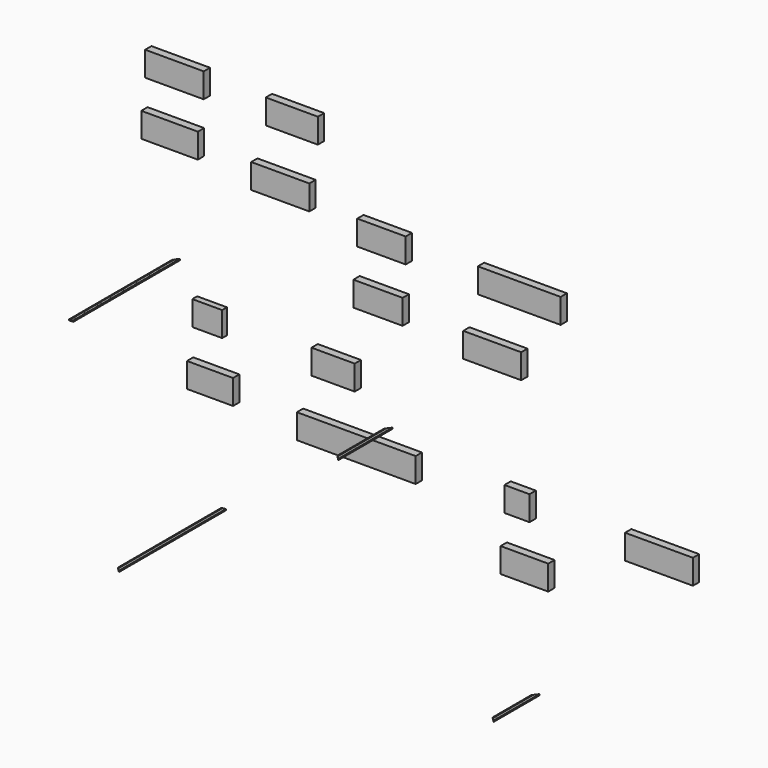
from build123d import *

# Parameters (mm, degrees)
F0_W        = 920.75
F0_H        = 387.35
F1_DEPTH    = 123.825
F0_W_2      = 889
F0_W_3      = 819.15
F0_W_4      = 914.4
F2_DEPTH    = 2101.85
F3_R        = 3.17499
F4_T1_DEPTH = 368.7891234188
F5_DEPTH    = 2101.85
F6_SIZE     = 69.84999
F0_W_5      = 762
F7_DEPTH    = 123.825
F0_W_6      = 1301.75
F0_W_7      = 774.7
F8_DEPTH    = 123.825
F0_W_8      = 911.225
F9_DEPTH    = 123.825
F0_W_9      = 679.45
F10_DEPTH   = 123.825
F0_W_10     = 469.9
F11_DEPTH   = 95.25
F0_W_11     = 723.9
F12_DEPTH   = 123.825
F0_W_12     = 1867.8652
F13_DEPTH   = 123.825
F0_W_13     = 393.7
F14_DEPTH   = 123.825
F0_W_14     = 1066.8
F15_DEPTH   = 123.825
F16_DEPTH   = 901.7
F17_SIZE    = 69.84999
F18_DEPTH   = 1060.45
F19_SIZE    = 69.84999
F0_W_15     = 749.3
F20_DEPTH   = 123.825


# Not quite as in the source:
# - a fillet or chamfer that OpenCascade refuses, or shapes differently, is made with other operations: its cross-section is extruded or revolved along the edge and cut away or added
# - a fillet or chamfer is up to 0.001 mm smaller than in the source, because OpenCascade refuses the exact size


with BuildPart() as f1:
    # F0 (on Front) → F1 (new body)
    with BuildSketch(Plane.XZ):
        with Locations((43.4228066687, 51.0344691575)):
            Rectangle(F0_W, F0_H)
    extrude(amount=F1_DEPTH)


with BuildPart() as f1b:
    # F0 (on Front) → F1, piece 2 (new body)
    with BuildSketch(Plane.XZ):
        with Locations((-33.3776168823, -813.8792926788)):
            Rectangle(F0_W_2, F0_H)
    extrude(amount=F1_DEPTH)


with BuildPart() as f1c:
    # F0 (on Front) → F1, piece 3 (new body)
    with BuildSketch(Plane.XZ):
        with Locations((1888.5462429047, 6.92840271)):
            Rectangle(F0_W_3, F0_H)
    extrude(amount=F1_DEPTH)


with BuildPart() as f1d:
    # F0 (on Front) → F1, piece 4 (new body)
    with BuildSketch(Plane.XZ):
        with Locations((1706.7899200439, -960.758965683)):
            Rectangle(F0_W_4, F0_H)
    extrude(amount=F1_DEPTH)


with BuildPart() as f2:
    # F0 (on Front) → F2 (new body)
    with BuildSketch(Plane.XZ):
        with BuildLine():
            Line((34.925, -2571.2136638563), (34.925, -2552.1636638563))
            Line((34.925, -2552.1636638563), (22.225, -2552.1636638563))
            Line((22.225, -2552.1636638563), (22.225, -2555.3386638563))
            add(Edge.make_bspline(
                [(22.225, -2555.3386638563), (14.0801436606, -2552.1636638563), (0.6341101832, -2556.6221824143), (-15.9369162842, -2556.0228194716), (-22.225, -2561.6886638563)],
                knots=[0, 0, 0, 0, 0.4950956813, 1, 1, 1, 1], degree=3))
            Line((-22.225, -2561.6886638563), (-22.225, -2558.5136638563))
            Line((-22.225, -2558.5136638563), (-34.925, -2558.5136638563))
            Line((-34.925, -2558.5136638563), (-34.925, -2571.2136638563))
            Line((-34.925, -2571.2136638563), (34.925, -2571.2136638563))
        make_face()
    extrude(amount=F2_DEPTH)

    # F3 (radius 3.175 in the source; OpenCascade refuses exactly that, so slightly less here)
    f3_edges = [f2.edges().sort_by_distance(p)[0] for p in [
        (-34.925, -1050.925, -2558.513664),
        (-22.225, -1050.925, -2558.513664),
        (22.225, -1050.925, -2552.163664),
        (34.925, -1050.925, -2552.163664),
    ]]
    fillet(f3_edges, radius=F3_R)

    # F4: chamfer of 69.85 on 1 edges, made by hand

    # F4_s2 → F4_t1 (cut)
    with BuildSketch(Plane.XY.offset(-2750.8457205657)):
        Polygon((34.925, 0), (-34.925, -69.85), (-34.925, 0), align=None)
    extrude(amount=F4_T1_DEPTH, mode=Mode.SUBTRACT)


with BuildPart() as f5:
    # F0 (on Front) → F5 (new body)
    with BuildSketch(Plane.XZ):
        with BuildLine():
            Line((753.253936991, -5800.0670439712), (753.253936991, -5781.0170439712))
            Line((753.253936991, -5781.0170439712), (740.553936991, -5781.0170439712))
            Line((740.553936991, -5781.0170439712), (740.553936991, -5784.1920439712))
            add(Edge.make_bspline(
                [(740.553936991, -5784.1920439712), (732.4090806516, -5781.0170439712), (718.9630471742, -5785.4755625292), (702.3920207068, -5784.8761995865), (696.103936991, -5790.5420439712)],
                knots=[0, 0, 0, 0, 0.4950956813, 1, 1, 1, 1], degree=3))
            Line((696.103936991, -5790.5420439712), (696.103936991, -5787.3670439712))
            Line((696.103936991, -5787.3670439712), (683.403936991, -5787.3670439712))
            Line((683.403936991, -5787.3670439712), (683.403936991, -5800.0670439712))
            Line((683.403936991, -5800.0670439712), (753.253936991, -5800.0670439712))
        make_face()
    extrude(amount=F5_DEPTH)

    # F6 (size 69.85 in the source; OpenCascade refuses exactly that, so slightly less here)
    f6_edges = [f5.edges().sort_by_distance(p)[0] for p in [
        (683.403937, -2101.85, -5793.717044),
    ]]
    chamfer(f6_edges, length=F6_SIZE)


with BuildPart() as f7:
    # F0 (on Front) → F7 (new body)
    with BuildSketch(Plane.XZ):
        with Locations((3297.7000487896, -1201.7320560228)):
            Rectangle(F0_W_5, F0_H)
    extrude(amount=F7_DEPTH)


with BuildPart() as f7b:
    # F0 (on Front) → F7, piece 2 (new body)
    with BuildSketch(Plane.XZ):
        with Locations((5463.4984850256, -1245.8381224703)):
            Rectangle(F0_W_6, F0_H)
    extrude(amount=F7_DEPTH)


with BuildPart() as f8:
    # F0 (on Front) → F8 (new body)
    with BuildSketch(Plane.XZ):
        with Locations((3243.1246252387, -2066.6458178591)):
            Rectangle(F0_W_7, F0_H)
    extrude(amount=F8_DEPTH)


with BuildPart() as f9:
    # F0 (on Front) → F9 (new body)
    with BuildSketch(Plane.XZ):
        with Locations((5038.8546621649, -2213.5254908632)):
            Rectangle(F0_W_8, F0_H)
    extrude(amount=F9_DEPTH)


with BuildPart() as f10:
    # F0 (on Front) → F10 (new body)
    with BuildSketch(Plane.XZ):
        with Locations((2537.0251798956, -3221.924977405)):
            Rectangle(F0_W_9, F0_H)
    extrude(amount=F10_DEPTH)


with BuildPart() as f11:
    # F0 (on Front) → F11 (new body)
    with BuildSketch(Plane.XZ):
        with Locations((536.3267436596, -3177.8189109575)):
            Rectangle(F0_W_10, F0_H)
    extrude(amount=F11_DEPTH)


with BuildPart() as f12:
    # F0 (on Front) → F12 (new body)
    with BuildSketch(Plane.XZ):
        with Locations((602.4013201087, -4042.7326727938)):
            Rectangle(F0_W_11, F0_H)
    extrude(amount=F12_DEPTH)


with BuildPart() as f13:
    # F0 (on Front) → F13 (new body)
    with BuildSketch(Plane.XZ):
        with Locations((2901.8514570349, -4189.6123457979)):
            Rectangle(F0_W_12, F0_H)
    extrude(amount=F13_DEPTH)


with BuildPart() as f14:
    # F0 (on Front) → F14 (new body)
    with BuildSketch(Plane.XZ):
        with Locations((5427.9554900738, -4135.6498168718)):
            Rectangle(F0_W_13, F0_H)
    extrude(amount=F14_DEPTH)


with BuildPart() as f15:
    # F0 (on Front) → F15 (new body)
    with BuildSketch(Plane.XZ):
        with Locations((7660.4289263098, -4179.7558833193)):
            Rectangle(F0_W_14, F0_H)
    extrude(amount=F15_DEPTH)


with BuildPart() as f16:
    # F0 (on Front) → F16 (new body)
    with BuildSketch(Plane.XZ):
        with BuildLine():
            Line((5682.9826834052, -6757.8979498855), (5682.9826834052, -6738.8479498855))
            Line((5682.9826834052, -6738.8479498855), (5670.2826834052, -6738.8479498855))
            Line((5670.2826834052, -6738.8479498855), (5670.2826834052, -6742.0229498855))
            add(Edge.make_bspline(
                [(5670.2826834052, -6742.0229498855), (5662.1378270658, -6738.8479498855), (5648.6917935884, -6743.3064684435), (5632.120767121, -6742.7071055008), (5625.8326834052, -6748.3729498855)],
                knots=[0, 0, 0, 0, 0.4950956813, 1, 1, 1, 1], degree=3))
            Line((5625.8326834052, -6748.3729498855), (5625.8326834052, -6745.1979498855))
            Line((5625.8326834052, -6745.1979498855), (5613.1326834052, -6745.1979498855))
            Line((5613.1326834052, -6745.1979498855), (5613.1326834052, -6757.8979498855))
            Line((5613.1326834052, -6757.8979498855), (5682.9826834052, -6757.8979498855))
        make_face()
    extrude(amount=F16_DEPTH)

    # F17 (size 69.85 in the source; OpenCascade refuses exactly that, so slightly less here)
    f17_edges = [f16.edges().sort_by_distance(p)[0] for p in [
        (5613.132683, -901.7, -6751.54795),
        (5613.132683, 0, -6751.54795),
    ]]
    chamfer(f17_edges, length=F17_SIZE)


with BuildPart() as f18:
    # F0 (on Front) → F18 (new body)
    with BuildSketch(Plane.XZ):
        with BuildLine():
            Line((3368.577242121, -3823.9801890365), (3368.577242121, -3804.9301890365))
            Line((3368.577242121, -3804.9301890365), (3355.877242121, -3804.9301890365))
            Line((3355.877242121, -3804.9301890365), (3355.877242121, -3808.1051890365))
            add(Edge.make_bspline(
                [(3355.877242121, -3808.1051890365), (3347.7323857816, -3804.9301890365), (3334.2863523042, -3809.3887075945), (3317.7153258368, -3808.7893446518), (3311.427242121, -3814.4551890365)],
                knots=[0, 0, 0, 0, 0.4950956813, 1, 1, 1, 1], degree=3))
            Line((3311.427242121, -3814.4551890365), (3311.427242121, -3811.2801890365))
            Line((3311.427242121, -3811.2801890365), (3298.727242121, -3811.2801890365))
            Line((3298.727242121, -3811.2801890365), (3298.727242121, -3823.9801890365))
            Line((3298.727242121, -3823.9801890365), (3368.577242121, -3823.9801890365))
        make_face()
    extrude(amount=F18_DEPTH)

    # F19 (size 69.85 in the source; OpenCascade refuses exactly that, so slightly less here)
    f19_edges = [f18.edges().sort_by_distance(p)[0] for p in [
        (3298.727242, -1060.45, -3817.630189),
        (3298.727242, 0, -3817.630189),
    ]]
    chamfer(f19_edges, length=F19_SIZE)


with BuildPart() as f20:
    # F0 (on Front) → F20 (new body)
    with BuildSketch(Plane.XZ):
        with Locations((5544.8300665228, -5000.5635787081)):
            Rectangle(F0_W_15, F0_H)
    extrude(amount=F20_DEPTH)


solid = Compound([f1.part, f1b.part, f1c.part, f1d.part, f2.part, f5.part, f7.part, f7b.part, f8.part, f9.part, f10.part, f11.part, f12.part, f13.part, f14.part, f15.part, f16.part, f18.part, f20.part])
